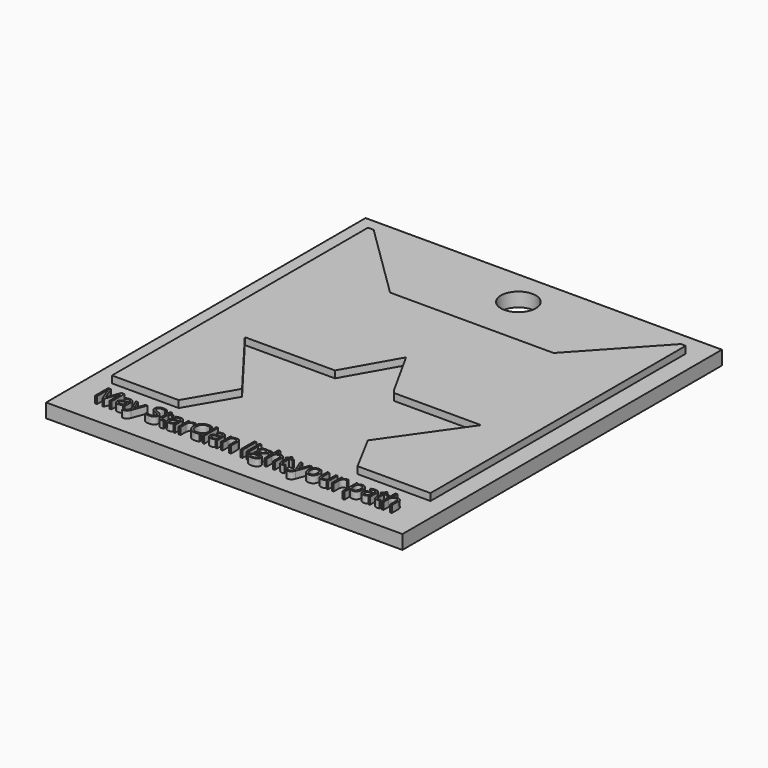
from build123d import *

# Parameters (mm, degrees)
F1_DEPTH     = 3
F2_W         = 51
F2_H         = 57.1551721228
F3_DEPTH     = 2
F5_D         = 5
F6_TEXT_SIZE = 3.2574455771
F7_DEPTH     = 1


# Not quite as in the source:
# - Text() gives the source's letters only with a copy of the font that has no kerning and outlines rounded to 1/6400 em; it was checked with that copy


with BuildPart() as f1:
    # F0 (on Top) → F1 (new body)
    with BuildSketch(Plane.XY):
        Polygon((2.8500626795, -1.7849690048), (2.0311151166, -1.7849690048), (2.0311151166, -47.5777760148), (11.5855010226, -47.5777760148), (15.4072558507, -41.0261973739), (7.8319925815, -31.0623366386), (20.7304134965, -31.0623366386), (24.9616410583, -23.6235652119), (28.7833958864, -30.5163711309), (29.2611159384, -31.1988275498), (41.7500622571, -31.1988275498), (34.1747999191, -41.9816337526), (37.1776074171, -47.5777760148), (47.6191863418, -47.5777760148), (47.6191863418, -1.9214592176), (46.9367280602, -1.9214592176), (37.1776074171, -12.4995298684), (13.7693611905, -12.4995298684), align=None)
    extrude(amount=F1_DEPTH)

    # F2 (on Top) → F3 (join)
    with BuildSketch(Plane.XY):
        with Locations((24.6650443296, -27.2023747675)):
            Rectangle(F2_W, F2_H)
    extrude(amount=F3_DEPTH)

    # F5 (through all)
    with Locations(Plane(origin=(0, 0, 0), x_dir=(1, 0, 0), z_dir=(0, 0, -1))):
        with Locations((25.1734051853, 3.7997590844)):
            Hole(F5_D / 2)

    # F6 (on face) → F7 (join)
    with BuildSketch(Plane.XY.offset(2)):
        with Locations((3.2957175281, -52.548840642)):
            Text('May StarClan light your path', F6_TEXT_SIZE, font='Open Sans', text_align=(TextAlign.LEFT, TextAlign.BOTTOM))
    extrude(amount=F7_DEPTH)


solid = f1.part
